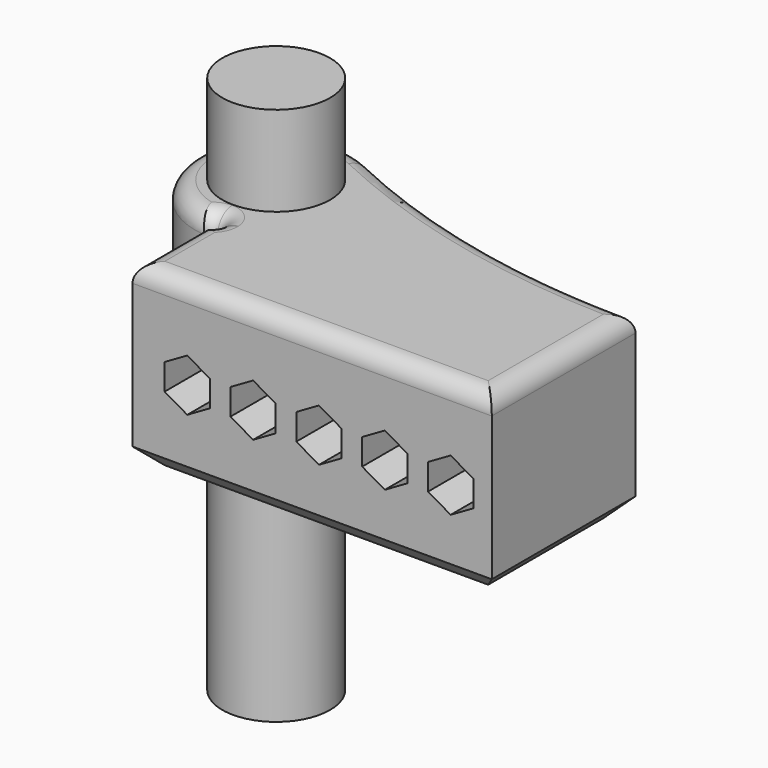
from build123d import *

# Parameters (mm, degrees)
F1_DEPTH = 50
F2_DEPTH = 75
F4_DEPTH = 72.501
F5_R     = 5
F6_SIZE  = 5


with BuildPart() as f1:
    # F0 (on Top) → F1 (new body)
    with BuildSketch(Plane.XY):
        with BuildLine():
            ThreePointArc((-52.0689964294, 11.0276228632), (-62.6755981472, 36.634224581), (-37.0689964294, 26.0276228632))
            Line((-37.0689964294, 26.0276228632), (-29.5689964294, 26.0276228632))
            ThreePointArc((-29.5689964294, 26.0276228632), (-33.0547226183, 38.0570613968), (-42.431875668, 46.3592706919))
            ThreePointArc((-42.431875668, 46.3592706919), (-73.7556932891, 32.0223855205), (-54.2425595338, 3.6328550942))
            ThreePointArc((-54.2425595338, 3.6328550942), (-53.5700716418, 5.103130273), (-52.0689964294, 5.7037318658))
            Line((-52.0689964294, 5.7037318658), (-52.0689964294, 11.0276228632))
        make_face()
        with BuildLine():
            Line((-29.5689964294, 26.0276228632), (-37.0689964294, 26.0276228632))
            ThreePointArc((-37.0689964294, 26.0276228632), (-41.4623947116, 15.4210211454), (-52.0689964294, 11.0276228632))
            Line((-52.0689964294, 11.0276228632), (-52.0689964294, 5.7037318658))
            ThreePointArc((-52.0689964294, 5.7037318658), (-50.5679212171, 5.103130273), (-49.8954333251, 3.6328550942))
            ThreePointArc((-49.8954333251, 3.6328550942), (-35.4083366309, 10.905704497), (-29.5689964294, 26.0276228632))
        make_face()
        with BuildLine():
            ThreePointArc((-42.431875668, 46.3592706919), (-33.0547226183, 38.0570613968), (-29.5689964294, 26.0276228632))
            Line((-29.5689964294, 26.0276228632), (47.9310035706, 26.0276228632))
            ThreePointArc((47.9310035706, 26.0276228632), (1.6200279608, 31.1732868199), (-42.431875668, 46.3592706919))
        make_face()
        with BuildLine():
            Line((47.9310035706, 26.0276228632), (-29.5689964294, 26.0276228632))
            ThreePointArc((-29.5689964294, 26.0276228632), (-35.4083366309, 10.905704497), (-49.8954333251, 3.6328550942))
            ThreePointArc((-49.8954333251, 3.6328550942), (-49.8935239945, 3.5802543748), (-49.8928874269, 3.5276228632))
            ThreePointArc((-49.8928874269, 3.5276228632), (-50.5302549971, 1.9888814309), (-52.0689964294, 1.3515138607))
            Line((-52.0689964294, 1.3515138607), (-52.0689964294, -23.9723771368))
            Line((-52.0689964294, -23.9723771368), (47.9310035706, -23.9723771368))
            Line((47.9310035706, -23.9723771368), (47.9310035706, 26.0276228632))
        make_face()
    extrude(amount=F1_DEPTH)

    # F3 (on face) → F4 (cut, through all)
    with BuildSketch(Plane.XZ.offset(23.9723771368)):
        Polygon((-30.5344704539, 21.364131914), (-30.5344704539, 28.635868086), (-36.8319787085, 32.2717361721), (-43.1294869632, 28.635868086), (-43.1294869632, 21.364131914), (-36.8319787085, 17.7282638279), align=None)
        Polygon((-18.5024917454, 32.1076042581), (-24.8, 28.4717361721), (-24.8, 21.2), (-18.5024917454, 17.564131914), (-12.2049834907, 21.2), (-12.2049834907, 28.4717361721), align=None)
        Polygon((-0.1730047822, 31.9434723442), (-6.4705130368, 28.3076042581), (-6.4705130368, 21.035868086), (-0.1730047822, 17.4), (6.1245034724, 21.035868086), (6.1245034724, 28.3076042581), align=None)
        Polygon((18.156482181, 31.7793404302), (11.8589739263, 28.1434723442), (11.8589739263, 20.8717361721), (18.156482181, 17.235868086), (24.4539904356, 20.8717361721), (24.4539904356, 28.1434723442), align=None)
        Polygon((36.4859691441, 31.6152085163), (30.1884608895, 27.9793404302), (30.1884608895, 20.7076042581), (36.4859691441, 17.0717361721), (42.7834773988, 20.7076042581), (42.7834773988, 27.9793404302), align=None)
    extrude(amount=-F4_DEPTH, mode=Mode.SUBTRACT)

    # F5
    f5_edges = [f1.edges().sort_by_distance(p)[0] for p in [
        (-2.068996, -23.972377, 50),
        (47.931004, 1.027623, 50),
        (1.620028, 31.173287, 50),
        (-73.755693, 32.022386, 50),
        (-52.068996, -11.310432, 50),
        (-50.493489, 5.028698, 50),
    ]]
    fillet(f5_edges, radius=F5_R)

    # F6
    f6_edges = [f1.edges().sort_by_distance(p)[0] for p in [
        (-2.068996, -23.972377, 0),
        (47.931004, 1.027623, 0),
        (1.620028, 31.173287, 0),
        (-73.755693, 32.022386, 0),
        (-50.493489, 5.028698, 0),
        (-52.068996, -11.310432, 0),
    ]]
    chamfer(f6_edges, length=F6_SIZE)


with BuildPart() as f2:
    # F0 (on Top) → F2 (new body, symmetric)
    with BuildSketch(Plane.XY):
        with BuildLine():
            Line((-37.0689964294, 26.0276228632), (-52.0689964294, 26.0276228632))
            Line((-52.0689964294, 26.0276228632), (-52.0689964294, 11.0276228632))
            ThreePointArc((-52.0689964294, 11.0276228632), (-41.4623947116, 15.4210211454), (-37.0689964294, 26.0276228632))
        make_face()
        with BuildLine():
            Line((-52.0689964294, 11.0276228632), (-52.0689964294, 26.0276228632))
            Line((-52.0689964294, 26.0276228632), (-37.0689964294, 26.0276228632))
            ThreePointArc((-37.0689964294, 26.0276228632), (-62.6755981472, 36.634224581), (-52.0689964294, 11.0276228632))
        make_face()
    extrude(amount=F2_DEPTH, both=True)


solid = Compound([f1.part, f2.part])
